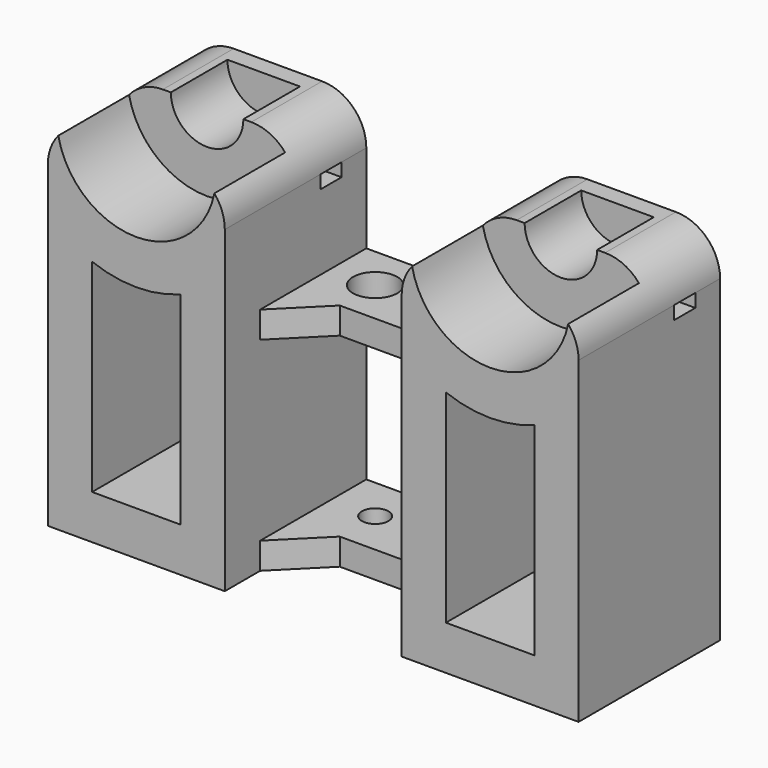
from build123d import *

# Parameters (mm, degrees)
F1_DEPTH  = 10
F2_W      = 14.1
F2_H      = 2
F3_DEPTH  = 10
F2_W_2    = 20
F5_DEPTH  = 10
F7_DEPTH  = 25
F8_W      = 3
F8_H      = 1.5
F9_DEPTH  = 100
F10_R     = 4.99999
F10_2_R   = 4.99999
F11_W     = 20
F11_H     = 3
F12_DEPTH = 10
F13_R     = 1.5
F14_DEPTH = 50
F15_R     = 2.5
F15_R_2   = 1.5
F16_DEPTH = 10
F17_SIZE  = 5


# Not quite as in the source:
# - a fillet or chamfer is up to 0.001 mm smaller than in the source, because OpenCascade refuses the exact size


with BuildPart() as f1:
    # F0 (on Front) → F1 (new body)
    with BuildSketch(Plane.XZ):
        with BuildLine():
            ThreePointArc((7, 0), (0, -7), (-7, 0))
            Line((-7, 0), (-10, 0))
            Line((-10, 0), (-10, -41))
            Line((-10, -41), (10, -41))
            Line((10, -41), (10, 0))
            Line((10, 0), (7, 0))
        make_face()
        with BuildLine():
            ThreePointArc((4.1, 0), (0, -4.1), (-4.1, 0))
            Line((-4.1, 0), (-7, 0))
            ThreePointArc((-7, 0), (0, -7), (7, 0))
            Line((7, 0), (4.1, 0))
        make_face()
    extrude(amount=F1_DEPTH)

    # F2 (on face) → F3 (join)
    with BuildSketch(Plane.XY):
        with Locations((2.95, -1)):
            Rectangle(F2_W, F2_H)
    extrude(amount=-F3_DEPTH)

    # F4 (on face) → F5 (join)
    with BuildSketch(Plane.XZ.offset(10)):
        with BuildLine():
            Line((10, 0), (9, 0))
            ThreePointArc((9, 0), (0, -9), (-9, 0))
            Line((-9, 0), (-10, 0))
            Line((-10, 0), (-10, -41))
            Line((-10, -41), (10, -41))
            Line((10, -41), (10, 0))
        make_face()
    extrude(amount=F5_DEPTH)


with BuildPart() as f1b:
    # F0 (on Front) → F1, piece 2 (new body)
    with BuildSketch(Plane.XZ):
        with BuildLine():
            Line((50, 0), (47, 0))
            ThreePointArc((47, 0), (40, -7), (33, 0))
            Line((33, 0), (30, 0))
            Line((30, 0), (30, -41))
            Line((30, -41), (50, -41))
            Line((50, -41), (50, 0))
        make_face()
        with BuildLine():
            ThreePointArc((33, 0), (40, -7), (47, 0))
            Line((47, 0), (44.1, 0))
            ThreePointArc((44.1, 0), (40, -4.1), (35.9, 0))
            Line((35.9, 0), (33, 0))
        make_face()
    extrude(amount=F1_DEPTH)

    # F2 (on face) → F3, piece 2 (join)
    with BuildSketch(Plane.XY):
        with Locations((40, -1)):
            Rectangle(F2_W_2, F2_H)
    extrude(amount=-F3_DEPTH)

    # F4 (on face) → F5, piece 2 (join)
    with BuildSketch(Plane.XZ.offset(10)):
        with BuildLine():
            Line((31, 0), (30, 0))
            Line((30, 0), (30, -41))
            Line((30, -41), (50, -41))
            Line((50, -41), (50, 0))
            Line((50, 0), (49, 0))
            ThreePointArc((49, 0), (40, -9), (31, 0))
        make_face()
    extrude(amount=F5_DEPTH)


with BuildPart() as f7_tool:
    # F6 (on face) → F7 (new body)
    with BuildSketch(Plane.XZ.offset(20)):
        with BuildLine():
            Line((5, -36), (5, -13.0766968306))
            ThreePointArc((5, -13.0766968306), (0, -14), (-5, -13.0766968306))
            Line((-5, -13.0766968306), (-5, -36))
            Line((-5, -36), (5, -36))
        make_face()
        with BuildLine():
            Line((45, -36), (45, -13.0766968306))
            ThreePointArc((45, -13.0766968306), (40, -14), (35, -13.0766968306))
            Line((35, -13.0766968306), (35, -36))
            Line((35, -36), (45, -36))
        make_face()
    extrude(amount=-F7_DEPTH)


with BuildPart() as f1_1:
    add(f1.part)

    # F7: cut by f7_tool
    add(f7_tool.part, mode=Mode.SUBTRACT)


with BuildPart() as f1b_1:
    add(f1b.part)

    # F7: cut by f7_tool
    add(f7_tool.part, mode=Mode.SUBTRACT)


with BuildPart() as f9_tool:
    # F8 (on face) → F9 (new body)
    with BuildSketch(Plane.YZ.offset(50)):
        with Locations((-5, -5.75)):
            Rectangle(F8_W, F8_H)
    extrude(amount=-F9_DEPTH)


with BuildPart() as f1_2:
    add(f1_1.part)

    # F9: cut by f9_tool
    add(f9_tool.part, mode=Mode.SUBTRACT)

    # F10#2 (radius 5 in the source; OpenCascade refuses exactly that, so slightly less here)
    f10_2_edges = [f1_2.edges().sort_by_distance(p)[0] for p in [
        (-10, -10, 0),
        (10, -10, 0),
    ]]
    fillet(f10_2_edges, radius=F10_2_R)



with BuildPart() as f1b_2:
    add(f1b_1.part)

    # F9: cut by f9_tool
    add(f9_tool.part, mode=Mode.SUBTRACT)

    # F10 (radius 5 in the source; OpenCascade refuses exactly that, so slightly less here)
    f10_edges = [f1b_2.edges().sort_by_distance(p)[0] for p in [
        (30, -10, 0),
        (50, -10, 0),
    ]]
    fillet(f10_edges, radius=F10_R)


with BuildPart() as f1_3:
    add(f1_2.part)

    add(f1b_2.part)  # F12 merges F1b
    # F11 (on face) → F12 (join)
    with BuildSketch(Plane(origin=(0, 0, 0), x_dir=(-1, 0, 0), z_dir=(0, 1, 0))):
        with Locations((-20, -39.5)):
            Rectangle(F11_W, F11_H)
        with Locations((-20, -16.5)):
            Rectangle(F11_W, F11_H)
    extrude(amount=-F12_DEPTH)

    # F13 (on face) → F14 (cut)
    with BuildSketch(Plane(origin=(0, 0, -41), x_dir=(1, 0, 0), z_dir=(0, 0, -1))):
        with Locations((15, 5)):
            Circle(F13_R)
        with Locations((25, 5)):
            Circle(F13_R)
    extrude(amount=-F14_DEPTH, mode=Mode.SUBTRACT)

    # F15 (on face) → F16 (cut)
    with BuildSketch(Plane.XY.offset(-15)):
        with Locations((15, -5)):
            Circle(F15_R)
        with Locations((15, -5)):
            Circle(F15_R_2, mode=Mode.SUBTRACT)
        with Locations((25, -5)):
            Circle(F15_R)
        with Locations((25, -5)):
            Circle(F15_R_2, mode=Mode.SUBTRACT)
    extrude(amount=-F16_DEPTH, mode=Mode.SUBTRACT)

    # F17
    f17_edges = [f1_3.edges().sort_by_distance(p)[0] for p in [
        (30, -10, -39.5),
        (10, -10, -39.5),
        (30, -10, -16.5),
        (10, -10, -16.5),
    ]]
    chamfer(f17_edges, length=F17_SIZE)


solid = f1_3.part
